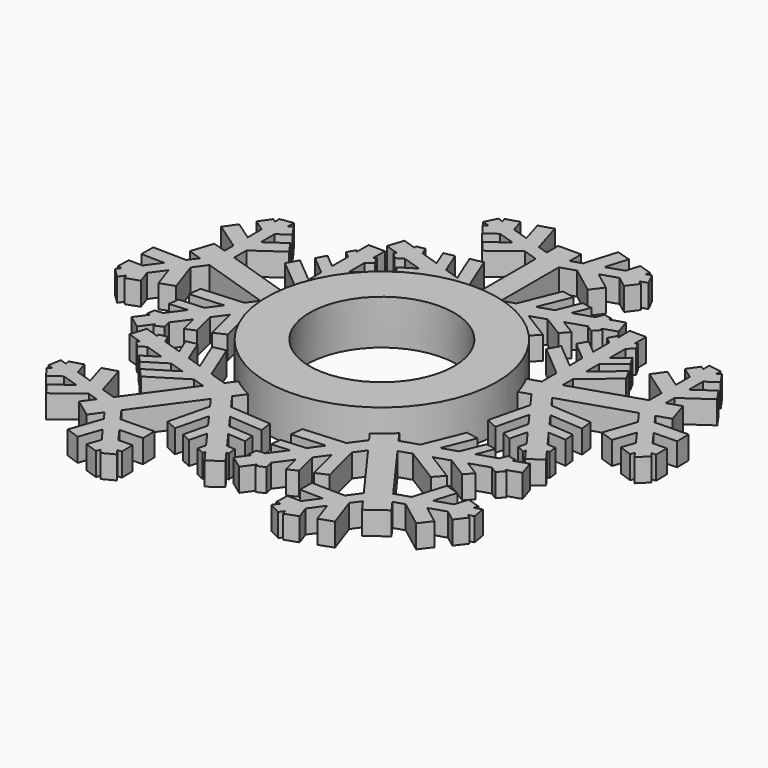
from build123d import *

# Parameters (mm, degrees)
F0_R            = 17.5
F1_DEPTH        = 7
F2_R            = 11
F3_DEPTH        = 7.001
F3_TAPER        = -3
F5_DEPTH        = 3.5
F5_COPIES_COUNT = 5


# Not quite as in the source:
# - a pattern or mirror of a feature is missing from the dataset's text; its kind, count and spacing are read off the source's solid


with BuildPart() as f1:
    # F0 (on Top) → F1 (new body)
    with BuildSketch(Plane.XY):
        Circle(F0_R)
    extrude(amount=F1_DEPTH)

    # F2 (on face) → F3 (cut, through all)
    with BuildSketch(Plane.XY.offset(7)):
        Circle(F2_R)
    extrude(amount=-F3_DEPTH, taper=F3_TAPER, mode=Mode.SUBTRACT)

    # F4 (on Top) → F5 (join)
    with BuildSketch(Plane.XY):
        Polygon((-2.87768274, 19.2298749643), (-2.87768274, 14.093211852), (0.62231726, 14.093211852), (0.62231726, 19.2298749643), (3.2716832825, 20.0932531174), (8.6547444437, 16.7525629445), (9.971564566, 18.171487464), (5.6342772446, 20.8631776934), (7.9418812897, 21.6151820982), (11.1314442991, 19.6357615636), (12.2198319642, 20.8085412916), (9.8946294916, 22.2515457119), (12.7821147688, 23.1925224152), (13.842731546, 22.5343110483), (14.743713735, 23.5051541406), (14.3986264271, 23.7193129146), (16.497272901, 24.4032220088), (15.7226638302, 26.7801908322), (13.6240173563, 26.096281738), (13.7766653754, 26.4726430176), (12.4766653754, 26.7262277465), (12.007505698, 25.5694912386), (9.1200204209, 24.6285145353), (10.1485646276, 27.1644414092), (8.5781629238, 27.4707720941), (7.167272219, 23.9921509216), (4.8596681738, 23.2401465168), (6.7782502328, 27.9705059622), (4.8782502328, 28.3411297968), (2.4970742117, 22.4702219408), (0.62231726, 21.8592741968), (0.62231726, 32.8710948533), (2.84288827, 33.5947368421), (6.8943460449, 30.532024347), (8.2391401494, 32.3109626375), (5.4269622322, 34.4368375508), (7.9567141202, 35.2612357254), (9.6530430197, 33.978890455), (10.9039966949, 35.6336935099), (10.3604700625, 36.0445742103), (11.4491937685, 36.3993686233), (10.5579747426, 38.189823495), (9.7474504237, 37.9256889875), (9.9445294249, 38.5779190216), (7.958771619, 39.1779391749), (7.3436944814, 37.1423505026), (4.8139425934, 36.317952328), (5.8336188745, 39.6925558701), (3.6988992255, 40.3375866021), (2.2298686312, 35.4758516193), (0.62231726, 34.9519811076), (0.62231726, 37.1423505026), (-2.87768274, 37.1423505026), (-2.87768274, 34.9519811076), (-4.4852341113, 35.4758516193), (-5.9542647055, 40.3375866021), (-8.0889843545, 39.6925558701), (-7.0693080735, 36.317952328), (-9.5990599615, 37.1423505026), (-10.2141370991, 39.1779391749), (-12.199894905, 38.5779190216), (-12.0028159037, 37.9256889875), (-12.8133402226, 38.189823495), (-13.7045592486, 36.3993686233), (-12.6158355425, 36.0445742103), (-13.1593621749, 35.6336935099), (-11.9084084998, 33.978890455), (-10.2120796003, 35.2612357254), (-7.6823277122, 34.4368375508), (-10.4945056295, 32.3109626375), (-9.149711525, 30.532024347), (-5.0982537501, 33.5947368421), (-2.87768274, 32.8710948533), (-2.87768274, 21.8592741968), (-4.7524396918, 22.4702219408), (-7.1336157129, 28.3411297968), (-9.0336157129, 27.9705059622), (-7.1150336539, 23.2401465168), (-9.422637699, 23.9921509216), (-10.8335284038, 27.4707720941), (-12.4039301077, 27.1644414092), (-11.3753859009, 24.6285145353), (-14.2628711781, 25.5694912386), (-14.7320308554, 26.7262277465), (-16.0320308554, 26.4726430176), (-15.8793828364, 26.096281738), (-17.9780293103, 26.7801908322), (-18.752638381, 24.4032220088), (-16.6539919071, 23.7193129146), (-16.999079215, 23.5051541406), (-16.0980970261, 22.5343110483), (-15.0374802489, 23.1925224152), (-12.1499949717, 22.2515457119), (-14.4751974442, 20.8085412916), (-13.3868097791, 19.6357615636), (-10.1972467698, 21.6151820982), (-7.8896427246, 20.8631776934), (-12.226930046, 18.171487464), (-10.9101099237, 16.7525629445), (-5.5270487625, 20.0932531174), align=None)
    f5 = extrude(amount=F5_DEPTH)

    # F5_copies: F5 ×5 about axis
    f5_copies_axis = Axis((0, 0, 0), (0, 0, 1))
    for i in range(1, F5_COPIES_COUNT):
        add(f5.rotate(f5_copies_axis, i * 360 / F5_COPIES_COUNT))


solid = f1.part
